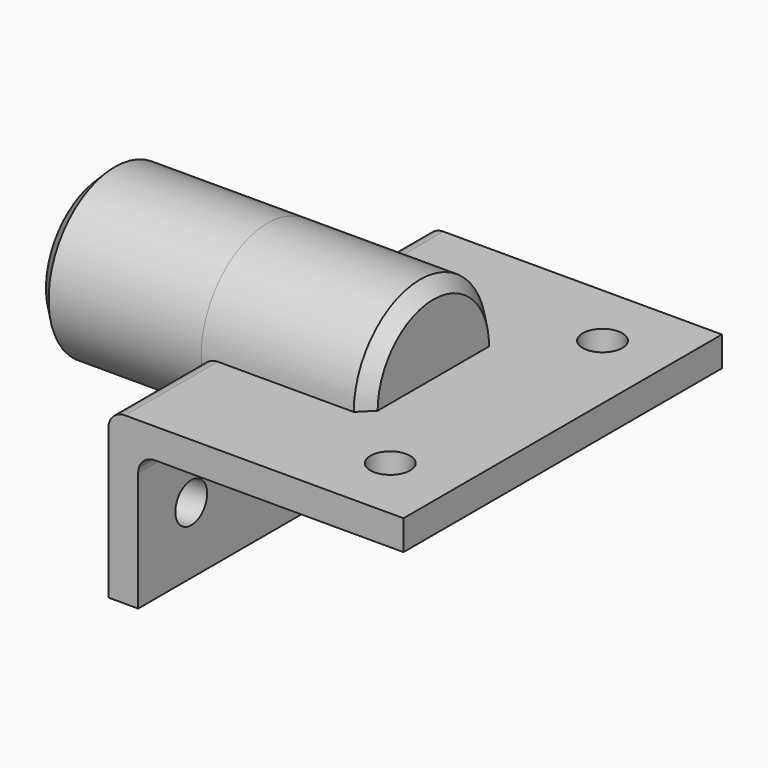
from build123d import *

# Parameters (mm, degrees)
F1_DEPTH      = 30
F2_R          = 12.5
F3_DEPTH      = 25
F3_DEPTH_BACK = 25
F4_SIZE       = 2
F5_R          = 3
F6_DEPTH      = 44.501
F7_R          = 3
F8_DEPTH      = 25.001


with BuildPart() as f1:
    # F0 (on Front) → F1 (new body, symmetric)
    with BuildSketch(Plane.XZ):
        with BuildLine():
            Line((44.5, 0), (2.5, 0))
            ThreePointArc((2.5, 0), (0.732233047, -0.732233047), (0, -2.5))
            Line((0, -2.5), (0, -25))
            Line((0, -25), (4.5, -25))
            Line((4.5, -25), (4.5, -7))
            ThreePointArc((4.5, -7), (5.232233047, -5.232233047), (7, -4.5))
            Line((7, -4.5), (44.5, -4.5))
            Line((44.5, -4.5), (44.5, 0))
        make_face()
    extrude(amount=F1_DEPTH, both=True)

    # F2 (on Right) → F3 (join, two sides)
    with BuildSketch(Plane.YZ) as f3_sk:
        Circle(F2_R)
    extrude(amount=F3_DEPTH)
    extrude(f3_sk.sketch, amount=-F3_DEPTH_BACK)

    # F4
    f4_edges = [f1.edges().sort_by_distance(p)[0] for p in [
        (-25, -12.5, 0),
        (25, 0, 12.5),
    ]]
    chamfer(f4_edges, length=F4_SIZE)

    # F5 (on face) → F6 (cut, through all)
    with BuildSketch(Plane(origin=(0, 0, 0), x_dir=(0, -1, 0), z_dir=(-1, 0, 0))):
        with Locations((-20, -15)):
            Circle(F5_R)
        with Locations((20, -15)):
            Circle(F5_R)
    extrude(amount=-F6_DEPTH, mode=Mode.SUBTRACT)

    # F7 (on face) → F8 (cut, through all)
    with BuildSketch(Plane.XY):
        with Locations((34.5, 20)):
            Circle(F7_R)
        with Locations((34.5, -20)):
            Circle(F7_R)
    extrude(amount=-F8_DEPTH, mode=Mode.SUBTRACT)


solid = f1.part
